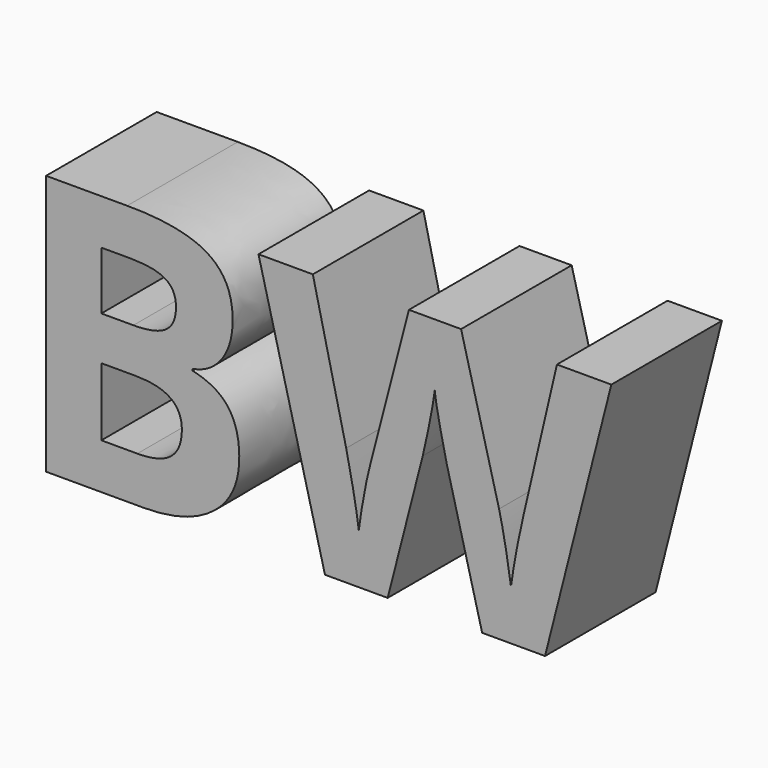
from build123d import *

# Parameters (mm, degrees)
F0_TEXT_SIZE = 66.0031843129
F1_DEPTH     = 25


# Not quite as in the source:
# - Text() gives the source's letters only with a copy of the font that has no kerning and outlines rounded to 1/6400 em; it was checked with that copy


with BuildPart() as f1:
    # F0 (on Front) → F1 (new body)
    with BuildSketch(Plane.XZ):
        with Locations((-12.850808911, -3.2090258319)):
            Text('BW', F0_TEXT_SIZE, font='Open Sans', font_style=FontStyle.BOLD, text_align=(TextAlign.LEFT, TextAlign.BOTTOM))
    extrude(amount=F1_DEPTH)


solid = f1.part
